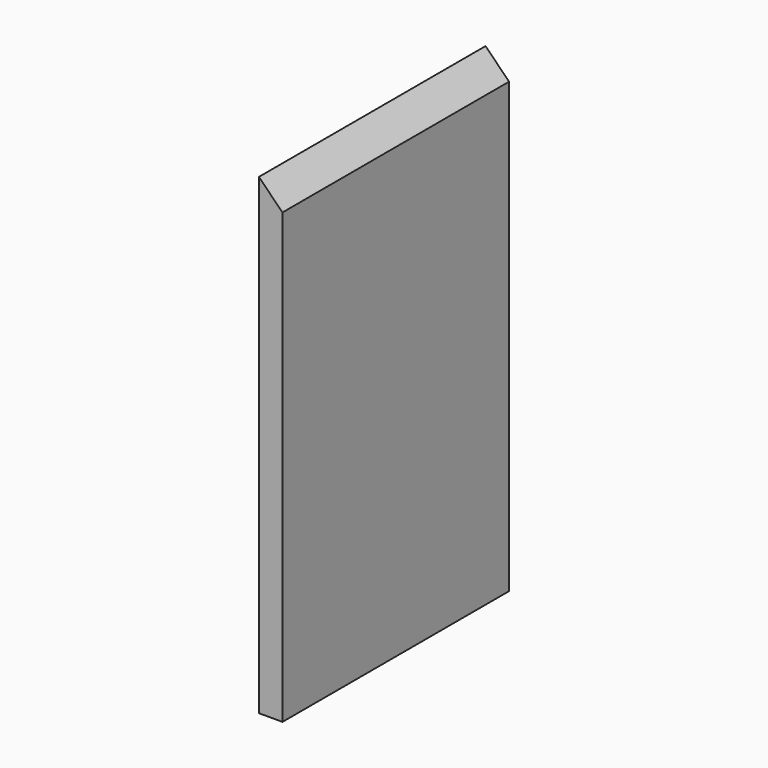
from build123d import *

# Parameters (mm, degrees)
F0_W     = 120
F0_H     = 200
F1_DEPTH = 10
F2_SIZE  = 9.99999


# Not quite as in the source:
# - a fillet or chamfer is up to 0.001 mm smaller than in the source, because OpenCascade refuses the exact size


with BuildPart() as f1:
    # F0 (on Right) → F1 (new body)
    with BuildSketch(Plane.YZ):
        Rectangle(F0_W, F0_H)
    extrude(amount=F1_DEPTH)

    # F2 (size 10 in the source; OpenCascade refuses exactly that, so slightly less here)
    f2_edges = [f1.edges().sort_by_distance(p)[0] for p in [
        (10, 0, 100),
    ]]
    chamfer(f2_edges, length=F2_SIZE)


solid = f1.part
